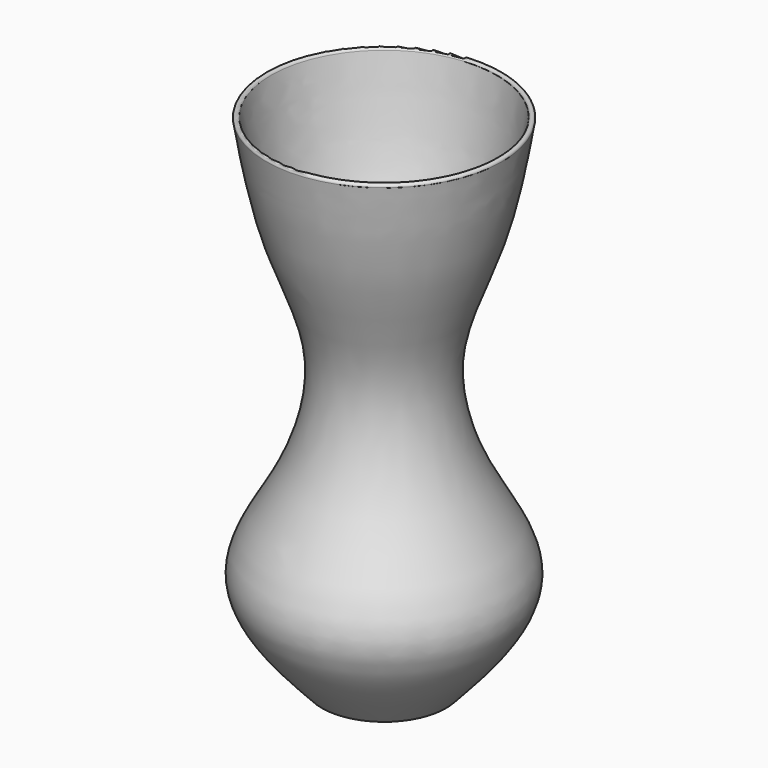
from build123d import *

# Parameters (mm, degrees)
F0_W = 5
F0_H = 5


# Not quite as in the source:
# - the dataset's text gives a spline's control points without its knots; the knots are read off the source's solid


with BuildPart() as f1:
    # F0 (on Front) → F1 (revolve)
    with BuildSketch(Plane.XZ):
        with Locations((-2.5, -2.5)):
            Rectangle(F0_W, F0_H)
        with BuildLine():
            Line((-5, 0), (0, 0))
            Line((0, 0), (0, 1.357470914))
            Line((0, 1.357470914), (-23.3744483674, 1.357470914))
            add(Edge.make_bspline(
                [(-23.3744483674, 1.357470914), (-26.9940154857, 5.2737950295), (-32.3958084194, 11.1202548003), (-38.5974229234, 18.7926259764), (-42.5116314376, 24.4556489393), (-44.9669979841, 29.0639255642), (-46.3444322656, 32.6570174613), (-47.0630238008, 35.2991638271), (-47.3851311152, 37.4556042958), (-47.467854793, 39.1551372252), (-47.4366323083, 40.8595593368), (-47.1942215666, 43.0021437734), (-46.4084964609, 46.4777528716), (-44.7494455682, 50.9296022978), (-41.9425063015, 56.4629071494), (-39.1797430833, 61.2488563048), (-36.8758309462, 65.2017700904), (-35.1421745504, 68.2347216488), (-33.4424405909, 71.3435440457), (-31.8232180061, 74.5333096422), (-30.3081094419, 77.7814715165), (-28.4329715862, 82.1847590127), (-26.3840449379, 87.8038869714), (-24.4643511316, 94.6720795313), (-23.1532010798, 101.6058999887), (-22.6268855428, 107.3891814457), (-22.582680222, 111.9876234078), (-22.746649479, 115.4155028738), (-23.1200882918, 118.8094501955), (-23.8715848452, 123.2649518512), (-25.2223949579, 128.7254103965), (-27.3116814834, 135.1410271419), (-29.6843531472, 141.4654830014), (-32.1605084683, 147.7416653668), (-34.1641158717, 152.9677291628), (-35.6434792171, 157.1615596431), (-37.0170688293, 161.3834372842), (-38.5585731614, 166.7317126547), (-40.1718090355, 173.241039345), (-41.5961972128, 179.8283087594), (-43.3064907395, 188.6937352088), (-44.4482058994, 195.4120485635), (-45.2109120928, 199.900629864)],
                knots=[1e-10, 1e-10, 1e-10, 1e-10, 0.0625000001, 0.0937500001, 0.1250000001, 0.1562500001, 0.1718750001, 0.1875000001, 0.2031250001, 0.2109375001, 0.2187500001, 0.2343750001, 0.2500000001, 0.2812500001, 0.3125000001, 0.3437500001, 0.3593750001, 0.3750000001, 0.3906250001, 0.4062500001, 0.4218750001, 0.4375000001, 0.46875, 0.5, 0.53125, 0.5625, 0.578125, 0.59375, 0.609375, 0.625, 0.65625, 0.6875, 0.71875, 0.75, 0.78125, 0.796875, 0.8125, 0.84375, 0.875, 0.90625, 0.9375, 1, 1, 1, 1], degree=3))
            ThreePointArc((-45.2109120928, 199.900629864), (-46.3643009514, 200.7189782866), (-47.182649374, 199.5655894279))
            add(Edge.make_bspline(
                [(-24.8432140797, 0), (-36.7985504643, 12.9355170555), (-59.6165920238, 37.6243385384), (-31.8855243353, 72.3349389124), (-19.2476756471, 116.8035249141), (-39.7897618973, 156.0579100961), (-44.7015869636, 184.964357082), (-47.182649374, 199.5655894279)],
                knots=[0, 0, 0, 0, 0.2064358802, 0.3940050152, 0.597500231, 0.7966892075, 1, 1, 1, 1], degree=3))
            Line((-24.8432140797, 0), (-5, 0))
        make_face()
    revolve(axis=Axis((0, 0, 100), (0, 0, 1)))


solid = f1.part
